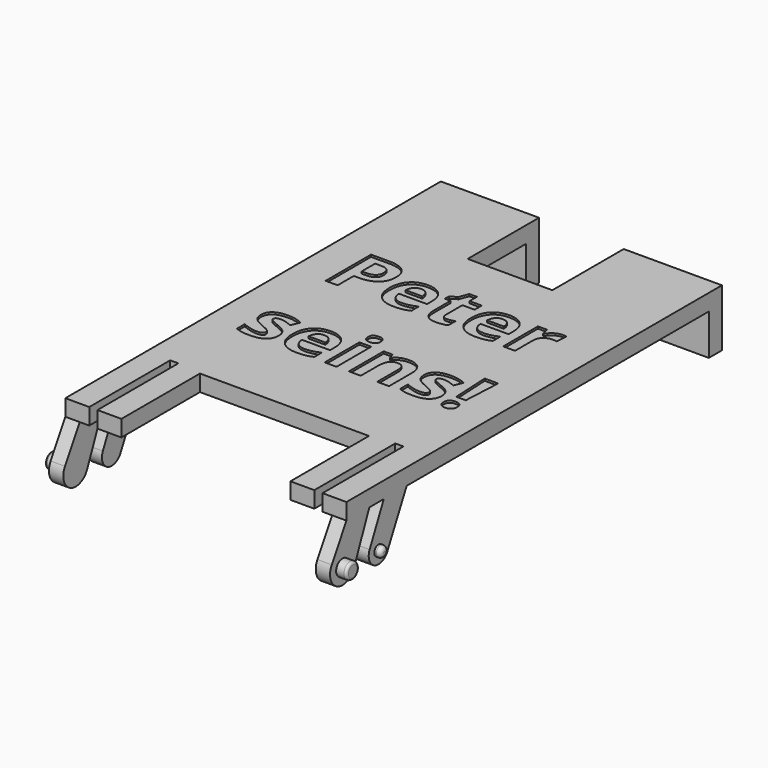
from build123d import *

# Parameters (mm, degrees)
F0_W          = 2
F0_H          = 2
F0_H_2        = 5
F0_W_2        = 55.35
F1_DEPTH      = 34.35
F2_W          = 20.65
F2_H          = 12.1
F2_W_2        = 10.35
F2_H_2        = 11
F2_W_3        = 1
F2_H_3        = 14.8744657636
F3_DEPTH      = 12.5
F5_DEPTH      = 1.75
F6_R          = 0.975
F7_DEPTH      = 1.25
F8_R          = 0.65
F9_DEPTH      = 0.75
F10_R         = 0.5
F11_R         = 0.3
F14_ANGLE     = 180
F15_TEXT_SIZE = 9.7222222222
F16_DEPTH     = 0.25


# Not quite as in the source:
# - Text() gives the source's letters only with a copy of the font that has no kerning and outlines rounded to 1/6400 em; it was checked with that copy


with BuildPart() as f1:
    # F0 (on Right) → F1 (new body)
    with BuildSketch(Plane.YZ):
        with Locations((24.0584141381, -1)):
            Rectangle(F0_W, F0_H)
        with Locations((24.0584141381, 2.5)):
            Rectangle(F0_W, F0_H_2)
        with Locations((-4.6165858619, -1)):
            Rectangle(F0_W_2, F0_H)
    extrude(amount=F1_DEPTH)

    # F2 (on Top) → F3 (cut, symmetric)
    with BuildSketch(Plane.XY):
        with Locations((17.175, -26.3415858619)):
            Rectangle(F2_W, F2_H)
        with Locations((17.175, 19.6584141381)):
            Rectangle(F2_W_2, F2_H_2)
        with Locations((3.425, -27.3714400828)):
            Rectangle(F2_W_3, F2_H_3)
        with Locations((30.925, -27.3714400828)):
            Rectangle(F2_W_3, F2_H_3)
    extrude(amount=F3_DEPTH, both=True, mode=Mode.SUBTRACT)



with BuildPart() as f5:
    # F4 (on Right) → F5 (new body)
    with BuildSketch(Plane.YZ):
        with BuildLine():
            ThreePointArc((-28.7476034845, 4.5587385813), (-27.062972437, 3.7364381745), (-25.8915858619, 5.2))
            ThreePointArc((-25.8915858619, 5.2), (-25.9322475599, 5.5468886282), (-26.0520281557, 5.8749704822))
            ThreePointArc((-26.0520281557, 5.8749704822), (-28.0497532695, 6.547893046), (-28.7476034845, 4.5587385813))
        make_face()
        with BuildLine():
            ThreePointArc((-26.0520281557, 5.8749704822), (-25.9322475599, 5.5468886282), (-25.8915858619, 5.2))
            ThreePointArc((-25.8915858619, 5.2), (-27.062972437, 3.7364381745), (-28.7476034845, 4.5587385813))
            Line((-28.7476034845, 4.5587385813), (-26.5917737067, 0))
            Line((-26.5917737067, 0), (-23.0917737067, 0))
            Line((-23.0917737067, 0), (-26.0520281557, 5.8749704822))
        make_face()
    extrude(amount=F5_DEPTH)


with BuildPart() as f5b:
    # F4 (on Right) → F5, piece 2 (new body)
    with BuildSketch(Plane.YZ):
        with BuildLine():
            ThreePointArc((-31.1424278606, 5.541920674), (-31.0296782108, 5.1785497309), (-30.9915858619, 4.8))
            ThreePointArc((-30.9915858619, 4.8), (-32.3958219989, 2.9658194767), (-34.5328681694, 3.8428206087))
            Line((-34.5328681694, 3.8428206087), (-32.2917737067, 0))
            Line((-32.2917737067, 0), (-28.7917737067, 0))
            Line((-28.7917737067, 0), (-31.1424278606, 5.541920674))
        make_face()
        with BuildLine():
            ThreePointArc((-34.5328681694, 3.8428206087), (-32.3958219989, 2.9658194767), (-30.9915858619, 4.8))
            ThreePointArc((-30.9915858619, 4.8), (-31.0296782108, 5.1785497309), (-31.1424278606, 5.541920674))
            ThreePointArc((-31.1424278606, 5.541920674), (-33.7428464267, 6.4986334068), (-34.5328681694, 3.8428206087))
        make_face()
    extrude(amount=F5_DEPTH)


with BuildPart() as f7:
    # F6 (on Right) → F7 (new body)
    with BuildSketch(Plane.YZ):
        with Locations((-32.8915858619, 4.8)):
            Circle(F6_R)
    extrude(amount=-F7_DEPTH)

    # F11
    f11_edges = [f7.edges().sort_by_distance(p)[0] for p in [
        (-1.25, -33.866586, 4.8),
    ]]
    fillet(f11_edges, radius=F11_R)


with BuildPart() as f9:
    # F8 (on Right) → F9 (new body)
    with BuildSketch(Plane.YZ):
        with Locations((-27.3915858619, 5.2)):
            Circle(F8_R)
    extrude(amount=-F9_DEPTH)

    # F10
    f10_edges = [f9.edges().sort_by_distance(p)[0] for p in [
        (-0.75, -28.041586, 5.2),
    ]]
    fillet(f10_edges, radius=F10_R)


with BuildPart() as f1_1:
    add(f1.part)

    add(f5.part)  # F13 merges F5

    add(f5b.part)  # F13 merges F5b

    add(f7.part)  # F13 merges F7

    add(f9.part)  # F13 merges F9
    # F13: F9, F5, F7, F5b across plane
    add(f9.part.mirror(Plane.YZ.offset(17.175)))
    add(f5.part.mirror(Plane.YZ.offset(17.175)))
    add(f7.part.mirror(Plane.YZ.offset(17.175)))
    add(f5b.part.mirror(Plane.YZ.offset(17.175)))


with BuildPart() as f1_2:
    # F14: moved
    add(f1_1.part.rotate(Axis((0, -0.0166797843, 0), (0, -1, 0)), F14_ANGLE))

    # F15 (on face) → F16 (cut, symmetric)
    with BuildSketch(Plane.XY.offset(2)):
        with Locations((-30.9805555556, 2.1584141381)):
            Text('Peter', F15_TEXT_SIZE, font='Open Sans', font_style=FontStyle.BOLD, text_align=(TextAlign.LEFT, TextAlign.BOTTOM))
        with Locations((-30.9805555556, -11.0638080841)):
            Text('seins!', F15_TEXT_SIZE, font='Open Sans', font_style=FontStyle.BOLD, text_align=(TextAlign.LEFT, TextAlign.BOTTOM))
    extrude(amount=F16_DEPTH, both=True, mode=Mode.SUBTRACT)


solid = f1_2.part
